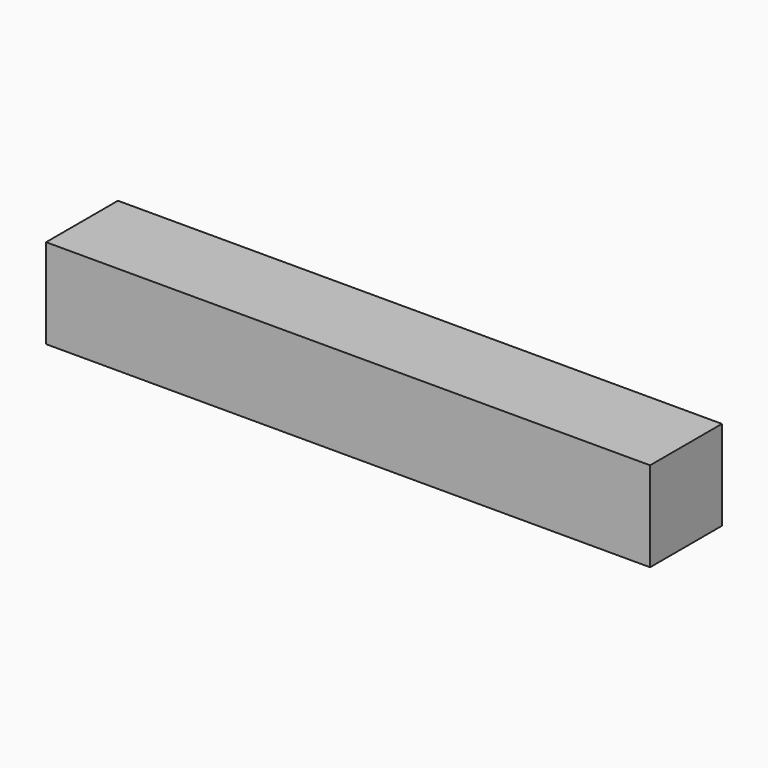
from build123d import *

# Parameters (mm, degrees)
F0_W     = 117.475
F0_H     = 17.4625
F1_DEPTH = 8.73125


# Not quite as in the source:
# - a length typed as a fraction of an inch, garbled in the dataset ("3 / 203.2 mm" for 3/8 in), is restored


with BuildPart() as f1:
    # F0 (on Front) → F1 (new body, symmetric)
    with BuildSketch(Plane.XZ):
        Rectangle(F0_W, F0_H)
    extrude(amount=F1_DEPTH, both=True)


solid = f1.part
